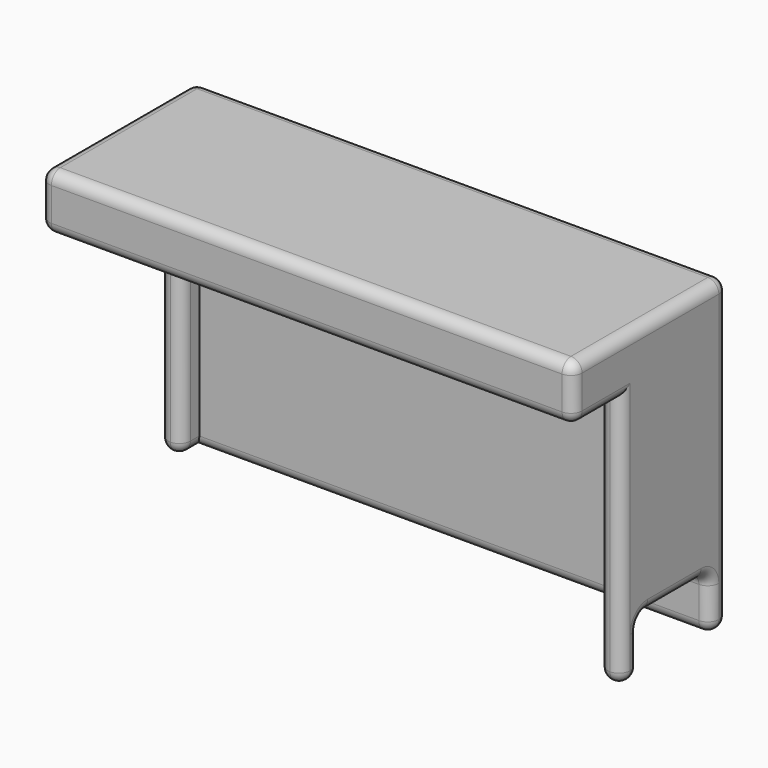
from build123d import *

# Parameters (mm, degrees)
F0_W     = 48
F0_H     = 27.8
F1_DEPTH = 2
F2_W     = 48
F2_H     = 2
F3_DEPTH = 15.4
F4_W     = 2
F4_H     = 10
F4_H_2   = 2
F5_DEPTH = 25.8
F7_DEPTH = 3
F8_W     = 8
F8_H     = 4.8617787947
F9_DEPTH = 2
F10_R    = 0.99999


# Not quite as in the source:
# - a fillet or chamfer is up to 0.001 mm smaller than in the source, because OpenCascade refuses the exact size


with BuildPart() as f1:
    # F0 (on Front) → F1 (new body)
    with BuildSketch(Plane.XZ):
        with Locations((24, 13.9)):
            Rectangle(F0_W, F0_H)
    extrude(amount=F1_DEPTH)

    # F2 (on face) → F3 (join)
    with BuildSketch(Plane.XZ.offset(2)):
        with Locations((24, 26.8)):
            Rectangle(F2_W, F2_H)
    extrude(amount=F3_DEPTH)

    # F4 (on face) → F5 (join)
    with BuildSketch(Plane(origin=(0, 0, 25.8), x_dir=(1, 0, 0), z_dir=(0, 0, -1))):
        with Locations((47, 7)):
            Rectangle(F4_W, F4_H)
        with Locations((1, 3)):
            Rectangle(F4_W, F4_H_2)
    extrude(amount=F5_DEPTH)

    # F6 (on face) → F7 (join)
    with BuildSketch(Plane(origin=(0, 0, 25.8), x_dir=(1, 0, 0), z_dir=(0, 0, -1))):
        Polygon((46, 15.4), (46, 12), (48, 12), (48, 17.4), (46, 17.4), (2, 17.4), (0, 17.4), (0, 4), (2, 4), (2, 15.4), align=None)
    extrude(amount=F7_DEPTH)

    # F8 (on face) → F9 (cut)
    with BuildSketch(Plane.YZ.offset(48)):
        with Locations((-6, 2.4308893974)):
            Rectangle(F8_W, F8_H)
    extrude(amount=-F9_DEPTH, mode=Mode.SUBTRACT)

    # F10 (radius 1 in the source; OpenCascade refuses exactly that, so slightly less here)
    f10_edges = [f1.edges().sort_by_distance(p)[0] for p in [
        (48, -8.7, 27.8),
        (24, -17.4, 27.8),
        (0, -8.7, 27.8),
        (24, 0, 27.8),
        (48, 0, 13.9),
        (48, -17.4, 25.3),
        (48, -14.7, 22.8),
        (48, -12, 11.4),
        (48, -11, 0),
        (48, -10, 2.430889),
        (48, -6, 4.861779),
        (48, -2, 2.430889),
        (48, -1, 0),
        (0, 0, 13.9),
        (24, 0, 0),
        (0, -17.4, 25.3),
        (24, -17.4, 22.8),
        (0, -10.7, 22.8),
        (0, -4, 11.4),
        (0, -2, 0),
        (47, -2, 4.861779),
        (47, -10, 4.861779),
        (46, -12, 11.4),
        (2, -4, 11.4),
        (2, -9.7, 22.8),
        (46, -13.7, 22.8),
        (24, -15.4, 22.8),
        (1, -4, 0),
        (25, -2, 0),
        (47, -10, 0),
        (46, -11, 0),
        (2, -3, 0),
        (47, -12, 0),
    ]]
    fillet(f10_edges, radius=F10_R)


solid = f1.part
